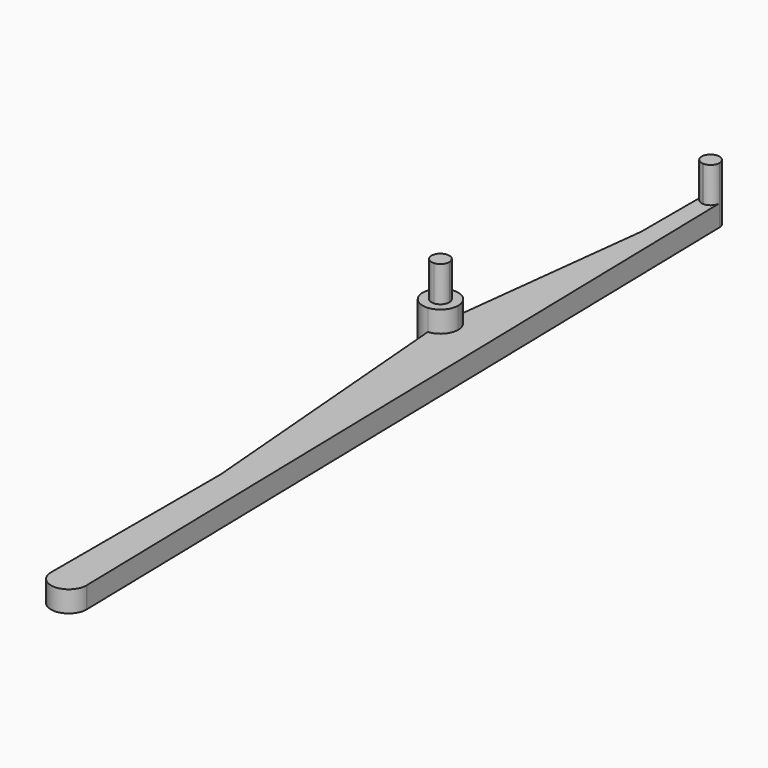
from build123d import *

# Parameters (mm, degrees)
F1_DEPTH = 6
F2_DEPTH = 11
F3_DEPTH = 8
F4_DEPTH = 3


# Not quite as in the source:
# - a feature names something its author has since deleted; it is built from what else it names


with BuildPart() as f1:
    # F0 (on Top) → F1 (new body)
    with BuildSketch(Plane.XY):
        with BuildLine():
            Line((48.7961772168, 43.654083433), (48.941615093, 44.8955937326))
            ThreePointArc((48.941615093, 44.8955937326), (46.1510840758, 42.4540888757), (48.8589984809, 39.9212626086))
            Line((48.8589984809, 39.9212626086), (48.7548689108, 41.1669178709))
            ThreePointArc((48.7548689108, 41.1669178709), (47.4009117082, 42.4333310045), (48.7961772168, 43.654083433))
        make_face()
        with BuildLine():
            ThreePointArc((51.1507393406, 42.4125731333), (50.5185173495, 44.0743208005), (48.941615093, 44.8955937326))
            Line((48.941615093, 44.8955937326), (48.7961772168, 43.654083433))
            ThreePointArc((48.7961772168, 43.654083433), (49.5846283451, 43.2434469669), (49.9007393406, 42.4125731333))
            ThreePointArc((49.9007393406, 42.4125731333), (49.5707018297, 41.5663054341), (48.7548689108, 41.1669178709))
            Line((48.7548689108, 41.1669178709), (48.8589984809, 39.9212626086))
            ThreePointArc((48.8589984809, 39.9212626086), (50.4906643188, 40.7200377349), (51.1507393406, 42.4125731333))
        make_face()
    extrude(amount=F1_DEPTH)

    # F0 (on Top) → F2 (join)
    with BuildSketch(Plane.XY):
        with BuildLine():
            ThreePointArc((49.9007393406, 42.4125731333), (49.5846283451, 43.2434469669), (48.7961772168, 43.654083433))
            Line((48.7961772168, 43.654083433), (48.6507393406, 42.4125731333))
            Line((48.6507393406, 42.4125731333), (48.7548689108, 41.1669178709))
            ThreePointArc((48.7548689108, 41.1669178709), (49.5707018297, 41.5663054341), (49.9007393406, 42.4125731333))
        make_face()
        with BuildLine():
            Line((48.6507393406, 42.4125731333), (48.7961772168, 43.654083433))
            ThreePointArc((48.7961772168, 43.654083433), (47.4009117082, 42.4333310045), (48.7548689108, 41.1669178709))
            Line((48.7548689108, 41.1669178709), (48.6507393406, 42.4125731333))
        make_face()
    extrude(amount=F2_DEPTH)



with BuildPart() as f3:
    # F0 (on Top) → F3 (new body)
    with BuildSketch(Plane.XY):
        with BuildLine():
            Line((53.5294346637, 82.6926567151), (53.515810825, 83.9425824693))
            Line((53.515810825, 83.9425824693), (53.3703729488, 82.7010721697))
            ThreePointArc((53.3703729488, 82.7010721697), (53.4497696251, 82.6943282645), (53.5294346637, 82.6926567151))
        make_face()
        with BuildLine():
            Line((53.3703729488, 82.7010721697), (53.515810825, 83.9425824693))
            Line((53.515810825, 83.9425824693), (53.5294346637, 82.6926567151))
            ThreePointArc((53.5294346637, 82.6926567151), (54.4044980024, 83.0635289438), (54.765810825, 83.9425824693))
            ThreePointArc((54.765810825, 83.9425824693), (54.7657365792, 83.9562063081), (54.7655138506, 83.9698285284))
            ThreePointArc((54.7655138506, 83.9698285284), (53.5021869863, 85.1925082235), (52.265810825, 83.9425824693))
            ThreePointArc((52.265810825, 83.9425824693), (52.5819218206, 83.1117086357), (53.3703729488, 82.7010721697))
        make_face()
    extrude(amount=F3_DEPTH)


with BuildPart() as f1_1:
    add(f1.part)

    add(f3.part)  # F4 merges F3
    # F0 (on Top) → F4 (join)
    with BuildSketch(Plane.XY):
        with BuildLine():
            ThreePointArc((54.765810825, 83.9425824693), (54.4044980024, 83.0635289438), (53.5294346637, 82.6926567151))
            Line((53.5294346637, 82.6926567151), (54.7385631476, -28.239428033))
            ThreePointArc((54.7385631476, -28.239428033), (56.5044417212, -28.9428490232), (57.2652168763, -30.6847874233))
            Line((57.2652168763, -30.6847874233), (54.7655138506, 83.9698285284))
            ThreePointArc((54.7655138506, 83.9698285284), (54.7657365792, 83.9562063081), (54.765810825, 83.9425824693))
        make_face()
        with BuildLine():
            Line((54.7385631476, -28.239428033), (53.5294346637, 82.6926567151))
            ThreePointArc((53.5294346637, 82.6926567151), (53.4497696251, 82.6943282645), (53.3703729488, 82.7010721697))
            Line((53.3703729488, 82.7010721697), (52.265810825, 73.2721304859))
            Line((52.265810825, 73.2721304859), (52.265810825, -0.8329027879))
            Line((52.265810825, -0.8329027879), (54.5575516847, -28.2479690167))
            ThreePointArc((54.5575516847, -28.2479690167), (54.6479800039, -28.2420579057), (54.7385631476, -28.239428033))
        make_face()
        with BuildLine():
            Line((52.265810825, 73.2721304859), (53.3703729488, 82.7010721697))
            ThreePointArc((53.3703729488, 82.7010721697), (52.5819218206, 83.1117086357), (52.265810825, 83.9425824693))
            Line((52.265810825, 83.9425824693), (52.265810825, 73.2721304859))
        make_face()
        with BuildLine():
            ThreePointArc((57.2652168763, -30.6847874233), (56.5044417212, -28.9428490232), (54.7385631476, -28.239428033))
            Line((54.7385631476, -28.239428033), (54.765810825, -30.7392795414))
            Line((54.765810825, -30.7392795414), (54.5575516847, -28.2479690167))
            ThreePointArc((54.5575516847, -28.2479690167), (52.9258858468, -29.0467441431), (52.265810825, -30.7392795414))
            ThreePointArc((52.265810825, -30.7392795414), (54.765810825, -33.2392795414), (57.265810825, -30.7392795414))
            ThreePointArc((57.265810825, -30.7392795414), (57.2656623334, -30.712031864), (57.2652168763, -30.6847874233))
        make_face()
        with BuildLine():
            Line((54.765810825, -30.7392795414), (54.7385631476, -28.239428033))
            ThreePointArc((54.7385631476, -28.239428033), (54.6479800039, -28.2420579057), (54.5575516847, -28.2479690167))
            Line((54.5575516847, -28.2479690167), (54.765810825, -30.7392795414))
        make_face()
        with BuildLine():
            Line((52.265810825, -0.8329027879), (52.265810825, 73.2721304859))
            Line((52.265810825, 73.2721304859), (48.941615093, 44.8955937326))
            ThreePointArc((48.941615093, 44.8955937326), (50.5185173495, 44.0743208005), (51.1507393406, 42.4125731333))
            ThreePointArc((51.1507393406, 42.4125731333), (50.4906643188, 40.7200377349), (48.8589984809, 39.9212626086))
            Line((48.8589984809, 39.9212626086), (52.265810825, -0.8329027879))
        make_face()
        with BuildLine():
            ThreePointArc((52.265810825, -30.7392795414), (52.9258858468, -29.0467441431), (54.5575516847, -28.2479690167))
            Line((54.5575516847, -28.2479690167), (52.265810825, -0.8329027879))
            Line((52.265810825, -0.8329027879), (52.265810825, -30.7392795414))
        make_face()
    extrude(amount=F4_DEPTH)


solid = f1_1.part
